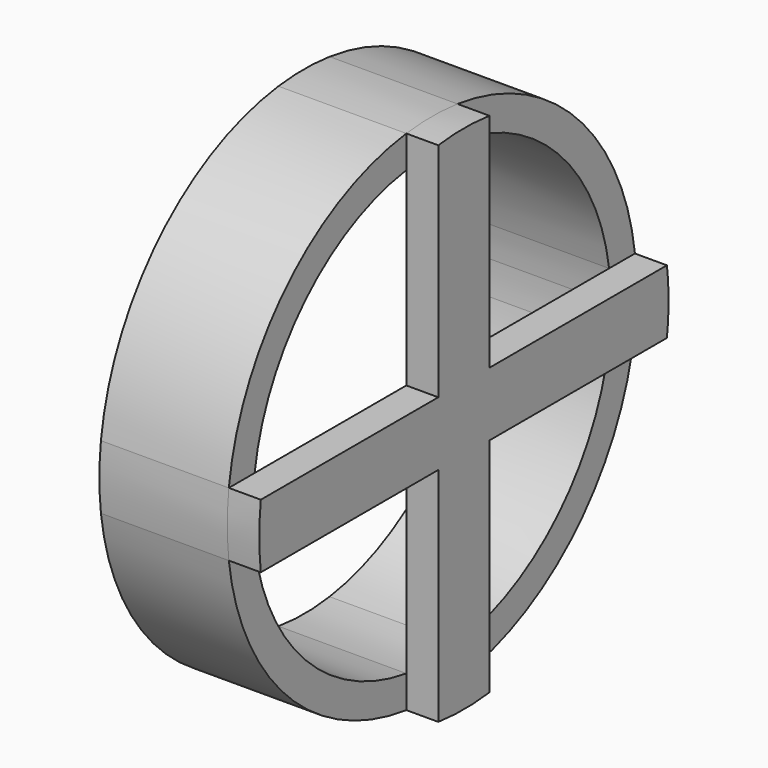
from build123d import *

# Parameters (mm, degrees)
F1_DEPTH = 6.3499999233
F2_DEPTH = 25.4


with BuildPart() as f1:
    # F0 (on Right) → F1 (new body)
    with BuildSketch(Plane.YZ):
        with BuildLine():
            Line((-5.5871092111, 47.5208675413), (-5.5871092111, 53.9283395048))
            ThreePointArc((-5.5871092111, 53.9283395048), (-11.9371092111, 54.326777029), (-18.2871092111, 53.9283395048))
            Line((-18.2871092111, 53.9283395048), (-18.2871092111, 47.5208675413))
            ThreePointArc((-18.2871092111, 47.5208675413), (-11.9371092111, 47.976777029), (-5.5871092111, 47.5208675413))
        make_face()
        with BuildLine():
            ThreePointArc((32.5128907889, 3.526777029), (32.3987669124, 6.7099497176), (32.0569813012, 9.876777029))
            Line((32.0569813012, 9.876777029), (-5.5871092111, 9.876777029))
            Line((-5.5871092111, 9.876777029), (-5.5871092111, 47.5208675413))
            ThreePointArc((-5.5871092111, 47.5208675413), (-11.9371092111, 47.976777029), (-18.2871092111, 47.5208675413))
            Line((-18.2871092111, 47.5208675413), (-18.2871092111, 9.876777029))
            Line((-18.2871092111, 9.876777029), (-55.9311997233, 9.876777029))
            ThreePointArc((-55.9311997233, 9.876777029), (-56.3871092111, 3.526777029), (-55.9311997233, -2.823222971))
            Line((-55.9311997233, -2.823222971), (-18.2871092111, -2.823222971))
            Line((-18.2871092111, -2.823222971), (-18.2871092111, -40.4673134832))
            ThreePointArc((-18.2871092111, -40.4673134832), (-11.9371092111, -40.923222971), (-5.5871092111, -40.4673134832))
            Line((-5.5871092111, -40.4673134832), (-5.5871092111, -2.823222971))
            Line((-5.5871092111, -2.823222971), (32.0569813012, -2.823222971))
            ThreePointArc((32.0569813012, -2.823222971), (32.3987669124, 0.3436043405), (32.5128907889, 3.526777029))
        make_face()
        with BuildLine():
            Line((-55.9311997233, 9.876777029), (-62.3386716869, 9.876777029))
            ThreePointArc((-62.3386716869, 9.876777029), (-62.7371092111, 3.526777029), (-62.3386716869, -2.823222971))
            Line((-62.3386716869, -2.823222971), (-55.9311997233, -2.823222971))
            ThreePointArc((-55.9311997233, -2.823222971), (-56.3871092111, 3.526777029), (-55.9311997233, 9.876777029))
        make_face()
        with BuildLine():
            ThreePointArc((38.4644532647, -2.823222971), (38.7631835581, 0.3455330718), (38.8628907889, 3.526777029))
            ThreePointArc((38.8628907889, 3.526777029), (38.7631835581, 6.7080209862), (38.4644532647, 9.876777029))
            Line((38.4644532647, 9.876777029), (32.0569813012, 9.876777029))
            ThreePointArc((32.0569813012, 9.876777029), (32.3987669124, 6.7099497176), (32.5128907889, 3.526777029))
            ThreePointArc((32.5128907889, 3.526777029), (32.3987669124, 0.3436043405), (32.0569813012, -2.823222971))
            Line((32.0569813012, -2.823222971), (38.4644532647, -2.823222971))
        make_face()
        with BuildLine():
            ThreePointArc((-18.2871092111, -46.8747854467), (-11.9371092111, -47.273222971), (-5.5871092111, -46.8747854467))
            Line((-5.5871092111, -46.8747854467), (-5.5871092111, -40.4673134832))
            ThreePointArc((-5.5871092111, -40.4673134832), (-11.9371092111, -40.923222971), (-18.2871092111, -40.4673134832))
            Line((-18.2871092111, -40.4673134832), (-18.2871092111, -46.8747854467))
        make_face()
    extrude(amount=F1_DEPTH)


with BuildPart() as f2:
    # F0 (on Right) → F2 (new body)
    with BuildSketch(Plane.YZ):
        with BuildLine():
            ThreePointArc((38.4644532647, -2.823222971), (38.7631835581, 0.3455330718), (38.8628907889, 3.526777029))
            ThreePointArc((38.8628907889, 3.526777029), (38.7631835581, 6.7080209862), (38.4644532647, 9.876777029))
            Line((38.4644532647, 9.876777029), (32.0569813012, 9.876777029))
            ThreePointArc((32.0569813012, 9.876777029), (32.3987669124, 6.7099497176), (32.5128907889, 3.526777029))
            ThreePointArc((32.5128907889, 3.526777029), (32.3987669124, 0.3436043405), (32.0569813012, -2.823222971))
            Line((32.0569813012, -2.823222971), (38.4644532647, -2.823222971))
        make_face()
        with BuildLine():
            Line((32.0569813012, 9.876777029), (38.4644532647, 9.876777029))
            ThreePointArc((38.4644532647, 9.876777029), (23.9839152732, 39.4478015133), (-5.5871092111, 53.9283395048))
            Line((-5.5871092111, 53.9283395048), (-5.5871092111, 47.5208675413))
            ThreePointArc((-5.5871092111, 47.5208675413), (19.4937872127, 34.9576734528), (32.0569813012, 9.876777029))
        make_face()
        with BuildLine():
            ThreePointArc((-5.5871092111, -46.8747854467), (23.9839152732, -32.3942474552), (38.4644532647, -2.823222971))
            Line((38.4644532647, -2.823222971), (32.0569813012, -2.823222971))
            ThreePointArc((32.0569813012, -2.823222971), (19.4937872127, -27.9041193947), (-5.5871092111, -40.4673134832))
            Line((-5.5871092111, -40.4673134832), (-5.5871092111, -46.8747854467))
        make_face()
        with BuildLine():
            Line((-5.5871092111, 47.5208675413), (-5.5871092111, 53.9283395048))
            ThreePointArc((-5.5871092111, 53.9283395048), (-11.9371092111, 54.326777029), (-18.2871092111, 53.9283395048))
            Line((-18.2871092111, 53.9283395048), (-18.2871092111, 47.5208675413))
            ThreePointArc((-18.2871092111, 47.5208675413), (-11.9371092111, 47.976777029), (-5.5871092111, 47.5208675413))
        make_face()
        with BuildLine():
            ThreePointArc((-18.2871092111, -46.8747854467), (-11.9371092111, -47.273222971), (-5.5871092111, -46.8747854467))
            Line((-5.5871092111, -46.8747854467), (-5.5871092111, -40.4673134832))
            ThreePointArc((-5.5871092111, -40.4673134832), (-11.9371092111, -40.923222971), (-18.2871092111, -40.4673134832))
            Line((-18.2871092111, -40.4673134832), (-18.2871092111, -46.8747854467))
        make_face()
        with BuildLine():
            Line((-18.2871092111, 47.5208675413), (-18.2871092111, 53.9283395048))
            ThreePointArc((-18.2871092111, 53.9283395048), (-47.8581336954, 39.4478015133), (-62.3386716869, 9.876777029))
            Line((-62.3386716869, 9.876777029), (-55.9311997233, 9.876777029))
            ThreePointArc((-55.9311997233, 9.876777029), (-43.3680056348, 34.9576734528), (-18.2871092111, 47.5208675413))
        make_face()
        with BuildLine():
            ThreePointArc((-62.3386716869, -2.823222971), (-47.8581336954, -32.3942474552), (-18.2871092111, -46.8747854467))
            Line((-18.2871092111, -46.8747854467), (-18.2871092111, -40.4673134832))
            ThreePointArc((-18.2871092111, -40.4673134832), (-43.3680056348, -27.9041193947), (-55.9311997233, -2.823222971))
            Line((-55.9311997233, -2.823222971), (-62.3386716869, -2.823222971))
        make_face()
        with BuildLine():
            Line((-55.9311997233, 9.876777029), (-62.3386716869, 9.876777029))
            ThreePointArc((-62.3386716869, 9.876777029), (-62.7371092111, 3.526777029), (-62.3386716869, -2.823222971))
            Line((-62.3386716869, -2.823222971), (-55.9311997233, -2.823222971))
            ThreePointArc((-55.9311997233, -2.823222971), (-56.3871092111, 3.526777029), (-55.9311997233, 9.876777029))
        make_face()
    extrude(amount=-F2_DEPTH)


solid = Compound([f1.part, f2.part])
